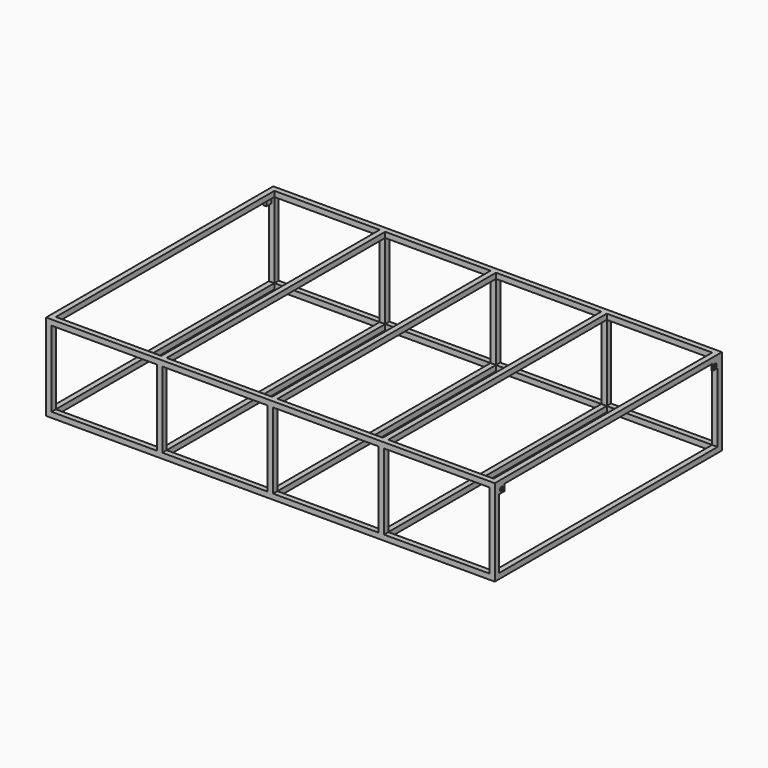
from build123d import *

# Parameters (mm, degrees)
F0_W      = 4140
F0_H      = 2620
F0_W_2    = 50
F0_H_2    = 2520
F1_DEPTH  = 50
F2_W      = 50
F2_H      = 50
F3_DEPTH  = 700
F7_W      = 2620
F7_H      = 800
F7_W_2    = 60
F7_H_2    = 60
F7_R      = 20
F8_DEPTH  = 10
F9_W      = 60
F9_H      = 60
F9_R      = 18.5
F10_DEPTH = 25
F11_DEPTH = 25
F12_R     = 7
F12_2_R   = 7


# Not quite as in the source:
# - a feature names something its author has since deleted; it is built from what else it names


with BuildPart() as f1:
    # F0 (on Top) → F1 (new body)
    with BuildSketch(Plane.XY):
        Rectangle(F0_W, F0_H)
        Polygon((1047.5, 1260), (2020, 1260), (2020, -1260), (1047.5, -1260), (997.5, -1260), (25, -1260), (-25, -1260), (-997.5, -1260), (-1047.5, -1260), (-2020, -1260), (-2020, 1260), (-1047.5, 1260), (-997.5, 1260), (-25, 1260), (25, 1260), (997.5, 1260), align=None, mode=Mode.SUBTRACT)
        with Locations((-1022.5, 0)):
            Rectangle(F0_W_2, F0_H_2)
        Rectangle(F0_W_2, F0_H_2)
        with Locations((1022.5, 0)):
            Rectangle(F0_W_2, F0_H_2)
    extrude(amount=-F1_DEPTH)

    # F2 (on face) → F3 (join)
    with BuildSketch(Plane.XY):
        with Locations((-2045, 1285)):
            Rectangle(F2_W, F2_H)
        with Locations((-1022.5, 1285)):
            Rectangle(F2_W, F2_H)
        with Locations((0, 1285)):
            Rectangle(F2_W, F2_H)
        with Locations((1022.5, 1285)):
            Rectangle(F2_W, F2_H)
        with Locations((2045, 1285)):
            Rectangle(F2_W, F2_H)
        with Locations((2045, -1285)):
            Rectangle(F2_W, F2_H)
        with Locations((1022.5, -1285)):
            Rectangle(F2_W, F2_H)
        with Locations((0, -1285)):
            Rectangle(F2_W, F2_H)
        with Locations((-1022.5, -1285)):
            Rectangle(F2_W, F2_H)
        with Locations((-2045, -1285)):
            Rectangle(F2_W, F2_H)
    extrude(amount=F3_DEPTH)

    # F6: F1 across plane


with BuildPart() as f1_1:
    add(f1.part)
    add(f1.part.mirror(Plane.XY.offset(350)))

    # F7 (on face) → F8 (join)
    with BuildSketch(Plane.YZ.offset(2070)):
        with Locations((0, 350)):
            Rectangle(F7_W, F7_H)
        Polygon((1200, 700), (1260, 700), (1260, 640), (1260, 0), (-1260, 0), (-1260, 640), (-1260, 700), (-1200, 700), align=None, mode=Mode.SUBTRACT)
        with Locations((1230, 670)):
            Rectangle(F7_W_2, F7_H_2)
        with Locations((1230, 670)):
            Circle(F7_R, mode=Mode.SUBTRACT)
        with Locations((-1230, 670)):
            Rectangle(F7_W_2, F7_H_2)
        with Locations((-1230, 670)):
            Circle(F7_R, mode=Mode.SUBTRACT)
    extrude(amount=-F8_DEPTH)


with BuildPart() as f10:
    # F9 (on face) → F10 (new body)
    with BuildSketch(Plane(origin=(-2070, 0, 0), x_dir=(0, -1, 0), z_dir=(-1, 0, 0))):
        with Locations((-1230, 670)):
            Rectangle(F9_W, F9_H)
        with Locations((-1230, 670)):
            Circle(F9_R, mode=Mode.SUBTRACT)
        with Locations((-1230, 670)):
            Circle(F9_R)
    extrude(amount=-F10_DEPTH)


with BuildPart() as f10b:
    # F9 (on face) → F10, piece 2 (new body)
    with BuildSketch(Plane(origin=(-2070, 0, 0), x_dir=(0, -1, 0), z_dir=(-1, 0, 0))):
        with Locations((1230, 670)):
            Rectangle(F9_W, F9_H)
        with Locations((1230, 670)):
            Circle(F9_R, mode=Mode.SUBTRACT)
        with Locations((1230, 670)):
            Circle(F9_R)
    extrude(amount=-F10_DEPTH)


with BuildPart() as f11:
    # F9 (on face) → F11 (new body)
    with BuildSketch(Plane(origin=(-2070, 0, 0), x_dir=(0, -1, 0), z_dir=(-1, 0, 0))):
        with Locations((-1230, 670)):
            Circle(F9_R)
    extrude(amount=F11_DEPTH)

    # F12
    f12_edges = [f11.edges().sort_by_distance(p)[0] for p in [
        (-2095, 1248.5, 670),
    ]]
    fillet(f12_edges, radius=F12_R)


with BuildPart() as f11b:
    # F9 (on face) → F11, piece 2 (new body)
    with BuildSketch(Plane(origin=(-2070, 0, 0), x_dir=(0, -1, 0), z_dir=(-1, 0, 0))):
        with Locations((1230, 670)):
            Circle(F9_R)
    extrude(amount=F11_DEPTH)

    # F12#2
    f12_2_edges = [f11b.edges().sort_by_distance(p)[0] for p in [
        (-2095, -1211.5, 670),
    ]]
    fillet(f12_2_edges, radius=F12_2_R)


solid = Compound([f1_1.part, f10.part, f10b.part, f11.part, f11b.part])
